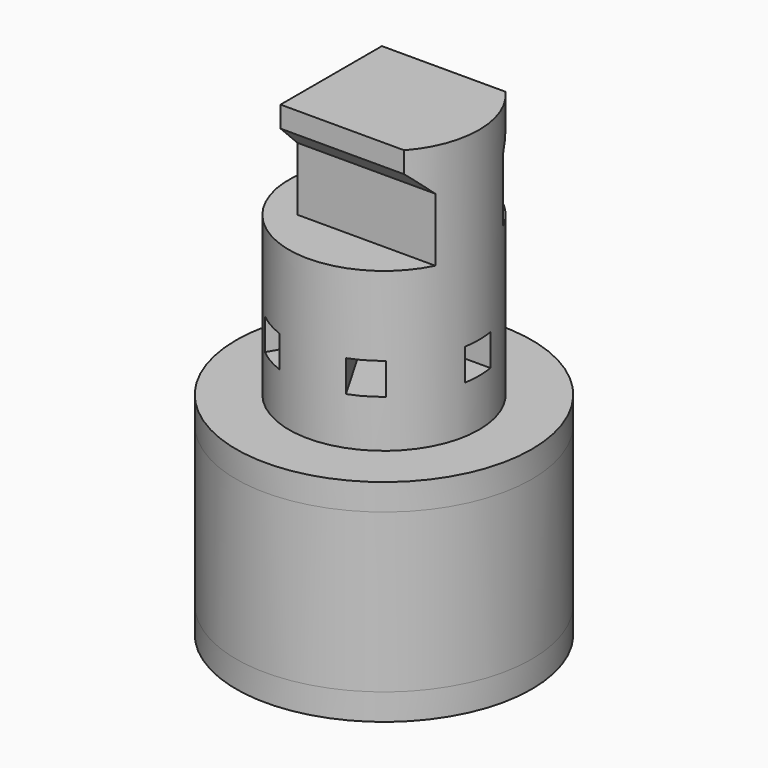
from build123d import *

# Parameters (mm, degrees)
F0_R          = 14
F0_R_2        = 12.5
F0_R_3        = 3.5
F0_R_4        = 2
F1_DEPTH      = 2.5
F2_DEPTH      = 15
F3_R          = 14
F3_R_2        = 2
F4_DEPTH      = 2.5
F5_R          = 9
F5_R_2        = 7.5
F5_R_3        = 3.5
F5_R_4        = 2
F6_DEPTH      = 25
F8_DEPTH      = 25
F8_DEPTH_BACK = 25
F9_W          = 8
F9_H          = 14.2362220213
F10_DEPTH     = 10
F11_DEPTH     = 25
F13_DEPTH     = 3
F14_DEPTH     = 2.5
F15_START     = 9.5
F15_DEPTH     = 2.5
F16_SIZE2     = 1.99999
F16_SIZE      = 1.99999


# Not quite as in the source:
# - a fillet or chamfer is up to 0.001 mm smaller than in the source, because OpenCascade refuses the exact size


with BuildPart() as f1:
    # F0 (on Top) → F1 (new body)
    with BuildSketch(Plane.XY):
        Circle(F0_R)
        Circle(F0_R_2, mode=Mode.SUBTRACT)
        Circle(F0_R_2)
        Circle(F0_R_3, mode=Mode.SUBTRACT)
        Circle(F0_R_3)
        Circle(F0_R_4, mode=Mode.SUBTRACT)
    extrude(amount=-F1_DEPTH)

    # F0 (on Top) → F2 (join)
    with BuildSketch(Plane.XY):
        Circle(F0_R)
        Circle(F0_R_2, mode=Mode.SUBTRACT)
        Circle(F0_R_3)
        Circle(F0_R_4, mode=Mode.SUBTRACT)
    extrude(amount=F2_DEPTH)

    # F3 (on face) → F4 (join)
    with BuildSketch(Plane.XY.offset(15)):
        Circle(F3_R)
        Circle(F3_R_2, mode=Mode.SUBTRACT)
    extrude(amount=F4_DEPTH)

    # F5 (on face) → F6 (join)
    with BuildSketch(Plane.XY.offset(17.5)):
        Circle(F5_R)
        Circle(F5_R_2, mode=Mode.SUBTRACT)
        Circle(F5_R_2)
        Circle(F5_R_3, mode=Mode.SUBTRACT)
        Circle(F5_R_3)
        Circle(F5_R_4, mode=Mode.SUBTRACT)
        Circle(F5_R_4)
    extrude(amount=F6_DEPTH)

    # F7 (on Right) → F8 (cut, two sides)
    with BuildSketch(Plane.YZ) as f8_sk:
        Polygon((-6, 40.5), (-6, 42.5), (-9, 42.5), (-9, 32.5), (-4, 32.5), (-4, 40.5), align=None)
        Polygon((9, 42.5), (6, 42.5), (6, 40.5), (4, 40.5), (4, 32.5), (9, 32.5), align=None)
    extrude(amount=F8_DEPTH, mode=Mode.SUBTRACT)
    extrude(f8_sk.sketch, amount=-F8_DEPTH_BACK, mode=Mode.SUBTRACT)

    # F9 (on face) → F10 (cut)
    with BuildSketch(Plane.XY.offset(42.5)):
        with Locations((-9, 0)):
            Rectangle(F9_W, F9_H)
    extrude(amount=-F10_DEPTH, mode=Mode.SUBTRACT)

    # F0 (on Top) → F11 (cut)
    with BuildSketch(Plane.XY):
        Circle(F0_R_4)
    extrude(amount=F11_DEPTH, mode=Mode.SUBTRACT)

    # F12 (on face) → F13 (cut)
    with BuildSketch(Plane(origin=(0, 0, 25), x_dir=(1, 0, 0), z_dir=(0, 0, -1))):
        Polygon((2.5980762114, -1.5), (23.6776883676, -1.5), (23.6776883676, 1.5), (2.5980762114, 1.5), (1.7320508076, 0), align=None)
        Polygon((13.1378822895, -19.7554796292), (2.5980762114, -1.5), (0.8660254038, -1.5), (0, -3), (10.5398060781, -21.2554796292), align=None)
        Polygon((0.8660254038, -1.5), (2.5980762114, -1.5), (1.7320508076, 0), align=None)
        Polygon((0, -3), (0.8660254038, -1.5), (-0.8660254038, -1.5), align=None)
        Polygon((0.8660254038, 1.5), (1.7320508076, 0), (2.5980762114, 1.5), align=None)
        Polygon((0.8660254038, 1.5), (2.5980762114, 1.5), (13.1378822895, 19.7554796292), (10.5398060781, 21.2554796292), (0, 3), align=None)
        Polygon((0, -3), (-0.8660254038, -1.5), (-2.5980762114, -1.5), (-13.1378822895, -19.7554796292), (-10.5398060781, -21.2554796292), align=None)
        Polygon((-2.5980762114, -1.5), (-0.8660254038, -1.5), (-1.7320508076, 0), align=None)
        Polygon((-0.8660254038, 1.5), (0.8660254038, 1.5), (0, 3), align=None)
        Polygon((-23.6776883676, -1.5), (-2.5980762114, -1.5), (-1.7320508076, 0), (-2.5980762114, 1.5), (-23.6776883676, 1.5), align=None)
        Polygon((-2.5980762114, 1.5), (-1.7320508076, 0), (-0.8660254038, 1.5), align=None)
        Polygon((-2.5980762114, 1.5), (-0.8660254038, 1.5), (0, 3), (-10.5398060781, 21.2554796292), (-13.1378822895, 19.7554796292), align=None)
    extrude(amount=F13_DEPTH, mode=Mode.SUBTRACT)

    # F5 (on face) → F14 (cut)
    with BuildSketch(Plane.XY.offset(17.5)):
        Circle(F5_R_2)
        Circle(F5_R_3, mode=Mode.SUBTRACT)
    extrude(amount=F14_DEPTH, mode=Mode.SUBTRACT)

    # F5 (on face) → F15 (cut)
    with BuildSketch(Plane.XY.offset(17.5).offset(F15_START)):
        Circle(F5_R_2)
        Circle(F5_R_3, mode=Mode.SUBTRACT)
    extrude(amount=F15_DEPTH, mode=Mode.SUBTRACT)

    # F16 (size 2 and 2 in the source; OpenCascade refuses exactly that, so slightly less here)
    f16_edges = [f1.edges().sort_by_distance(p)[0] for p in [
        (1.531129, -4, 40.5),
        (1.531129, 4, 40.5),
    ]]
    chamfer(f16_edges, length=F16_SIZE, length2=F16_SIZE2)


solid = f1.part
